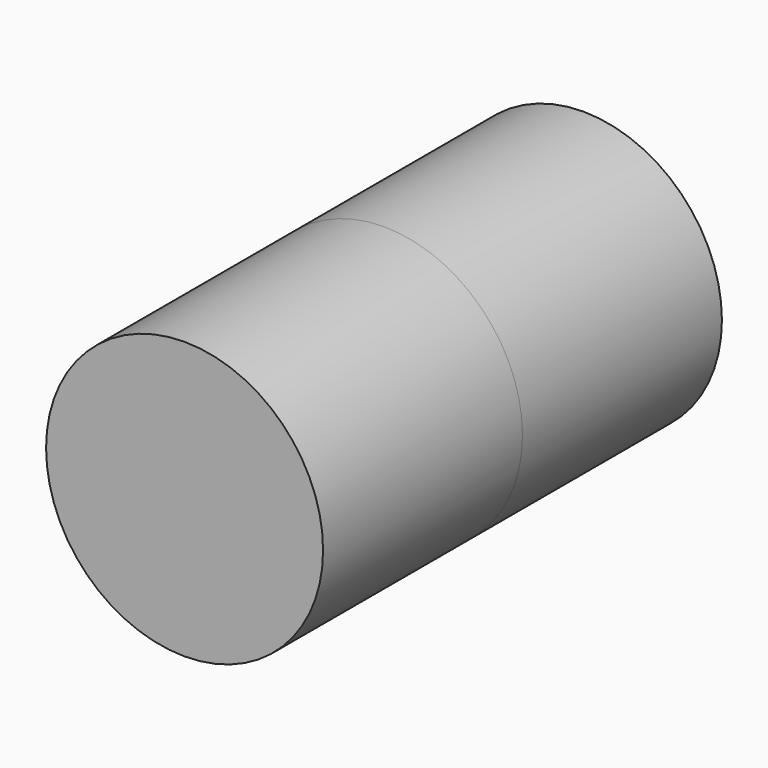
from build123d import *

# Parameters (mm, degrees)
F1_DEPTH = 135
F2_DEPTH = 135


# Not quite as in the source:
# - the program builds the solid bodies; features that only make, move or delete a surface that nothing else refers to are left out


with BuildPart() as f1:
    # F0 (on Front) → F1 (new body)
    with BuildSketch(Plane.XZ):
        with BuildLine():
            ThreePointArc((0, -75), (53.033008589, -53.033008589), (75, 0))
            ThreePointArc((75, 0), (53.033008589, 53.033008589), (0, 75))
            Line((0, 75), (0, -75))
        make_face()
        with BuildLine():
            Line((0, -75), (0, 75))
            ThreePointArc((0, 75), (-75, 0), (0, -75))
        make_face()
    extrude(amount=-F1_DEPTH)

    # F2 (add): a face of the model
    f2_faces = [f1.faces().sort_by_distance(p)[0] for p in [
        (0, 0, 0),
    ]]
    extrude(f2_faces, amount=F2_DEPTH)


solid = f1.part
